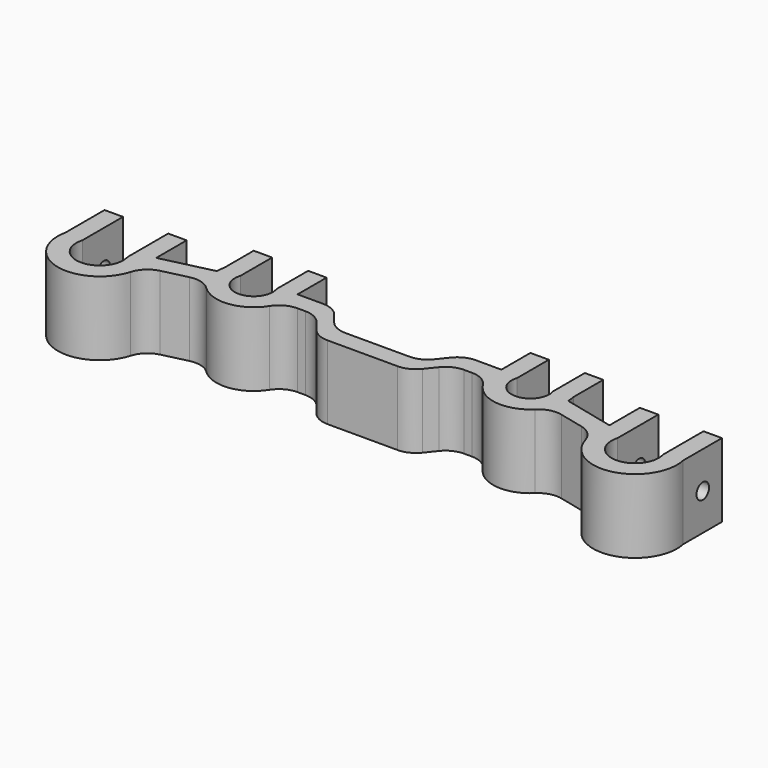
from build123d import *

# Parameters (mm, degrees)
F1_DEPTH = 16
F2_R     = 1.7
F3_DEPTH = 15.8
F4_DEPTH = 2
F5_R     = 1.7
F6_DEPTH = 17.8
F7_DEPTH = 2
F8_R     = 5


# Not quite as in the source:
# - a feature names something its author has since deleted; it is built from what else it names


with BuildPart() as f1:
    # F0 (on Top) → F1 (new body)
    with BuildSketch(Plane.XY):
        with BuildLine():
            ThreePointArc((-26.1, 1.2649110641), (-30, -4.1), (-33.9, 1.2649110641))
            Line((-33.9, 1.2649110641), (-33.9, 7.0992957397))
            ThreePointArc((-33.9, 7.0992957397), (-36.4699456608, 4.8733769756), (-37.9, 1.788854382))
            ThreePointArc((-37.9, 1.788854382), (-38.0425692419, 0.9628499311), (-38.0990116086, 0.1265344399))
            ThreePointArc((-38.0990116086, 0.1265344399), (-37.8794890645, -1.8771393349), (-37.1720292209, -3.7645712709))
            ThreePointArc((-37.1720292209, -3.7645712709), (-29.054976567, -8.0446833817), (-22.1507962187, -2))
            ThreePointArc((-22.1507962187, -2), (-21.9, 0), (-22.1507962187, 2))
            ThreePointArc((-22.1507962187, 2), (-23.5959659875, 4.9596722035), (-26.1, 7.0992957397))
            Line((-26.1, 7.0992957397), (-26.1, 1.2649110641))
        make_face()
        with BuildLine():
            ThreePointArc((-37.9, 1.788854382), (-36.4699456608, 4.8733769756), (-33.9, 7.0992957397))
            Line((-33.9, 7.0992957397), (-33.9, 9.8649110641))
            Line((-33.9, 9.8649110641), (-37.9, 9.8649110641))
            Line((-37.9, 9.8649110641), (-37.9, 1.788854382))
        make_face()
        with BuildLine():
            Line((-26.1, 9.8649110641), (-26.1, 7.0992957397))
            ThreePointArc((-26.1, 7.0992957397), (-23.5959659875, 4.9596722035), (-22.1507962187, 2))
            Line((-22.1507962187, 2), (-22.1, 2))
            Line((-22.1, 2), (-22.1, 9.8649110641))
            Line((-22.1, 9.8649110641), (-26.1, 9.8649110641))
        make_face()
        with BuildLine():
            Line((-22.1, 2), (-22.1507962187, 2))
            ThreePointArc((-22.1507962187, 2), (-21.9, 0), (-22.1507962187, -2))
            Line((-22.1507962187, -2), (-16.1507962187, -2))
            Line((-16.1507962187, -2), (-14.7945886775, -2))
            Line((-14.7945886775, -2), (-10, -8))
            Line((-10, -8), (0, -8))
            Line((0, -8), (0, -4))
            Line((0, -4), (-6, -4))
            Line((-6, -4), (-9.3562075412, -4))
            Line((-9.3562075412, -4), (-14.1507962187, 2))
            Line((-14.1507962187, 2), (-22.1, 2))
        make_face()
        with BuildLine():
            ThreePointArc((-37.1720292209, -3.7645712709), (-37.8794890645, -1.8771393349), (-38.0990116086, 0.1265344399))
            Line((-38.0990116086, 0.1265344399), (-49.14, -2.5037723523))
            Line((-49.14, -2.5037723523), (-49.14, -4.7826334039))
            ThreePointArc((-49.14, -4.7826334039), (-48.9961671585, -5.6705013446), (-48.9406864116, -6.5682314005))
            Line((-48.9406864116, -6.5682314005), (-37.1720292209, -3.7645712709))
        make_face()
        with BuildLine():
            Line((-49.14, -4.7826334039), (-49.14, -2.5037723523))
            Line((-49.14, -2.5037723523), (-49.8676687992, -2.6771256897))
            ThreePointArc((-49.8676687992, -2.6771256897), (-49.4391620268, -3.7075286109), (-49.14, -4.7826334039))
        make_face()
        with BuildLine():
            Line((-49.8676687992, -2.6771256897), (-49.14, -2.5037723523))
            Line((-49.14, -2.5037723523), (-49.14, 5.7342135624))
            Line((-49.14, 5.7342135624), (-53.14, 5.7342135624))
            Line((-53.14, 5.7342135624), (-53.14, 0.9881158051))
            ThreePointArc((-53.14, 0.9881158051), (-51.2517778793, -0.6194686338), (-49.8676687992, -2.6771256897))
        make_face()
        with BuildLine():
            ThreePointArc((-66.94, -4.7826334039), (-58.9383437694, -15.7355495952), (-48.9406864116, -6.5682314005))
            ThreePointArc((-48.9406864116, -6.5682314005), (-48.9961671585, -5.6705013446), (-49.14, -4.7826334039))
            ThreePointArc((-49.14, -4.7826334039), (-49.4391620268, -3.7075286109), (-49.8676687992, -2.6771256897))
            ThreePointArc((-49.8676687992, -2.6771256897), (-51.2517778793, -0.6194686338), (-53.14, 0.9881158051))
            Line((-53.14, 0.9881158051), (-53.14, -5.2657864376))
            ThreePointArc((-53.14, -5.2657864376), (-58.04, -11.78), (-62.94, -5.2657864376))
            Line((-62.94, -5.2657864376), (-62.94, 0.9881158051))
            ThreePointArc((-62.94, 0.9881158051), (-65.5189963637, -1.4959269496), (-66.94, -4.7826334039))
        make_face()
        with BuildLine():
            Line((-66.94, 5.7342135624), (-66.94, -4.7826334039))
            ThreePointArc((-66.94, -4.7826334039), (-65.5189963637, -1.4959269496), (-62.94, 0.9881158051))
            Line((-62.94, 0.9881158051), (-62.94, 5.7342135624))
            Line((-62.94, 5.7342135624), (-66.94, 5.7342135624))
        make_face()
    extrude(amount=F1_DEPTH)

    # F2 (on face) → F3 (cut, through all)
    with BuildSketch(Plane.YZ.offset(-22.1)):
        with Locations((5.2649110641, 8)):
            Circle(F2_R)
    extrude(amount=-F3_DEPTH, mode=Mode.SUBTRACT)

    # F2 (on face) → F4 (cut)
    with BuildSketch(Plane.YZ.offset(-22.1)):
        Polygon((8.1149110641, 6.3545517328), (8.1149110641, 9.6454482672), (5.2649110641, 11.2908965344), (2.4149110641, 9.6454482672), (2.4149110641, 6.3545517328), (5.2649110641, 4.7091034656), align=None)
        with Locations((5.2649110641, 8)):
            Circle(F2_R, mode=Mode.SUBTRACT)
    extrude(amount=-F4_DEPTH, mode=Mode.SUBTRACT)

    # F5 (on face) → F6 (cut, through all)
    with BuildSketch(Plane.YZ.offset(-49.14)):
        with Locations((0.5462276477, 8)):
            Circle(F5_R)
    extrude(amount=-F6_DEPTH, mode=Mode.SUBTRACT)

    # F5 (on face) → F7 (cut)
    with BuildSketch(Plane.YZ.offset(-49.14)):
        Polygon((3.3962276477, 6.3545517328), (3.3962276477, 9.6454482672), (0.5462276477, 11.2908965344), (-2.3037723523, 9.6454482672), (-2.3037723523, 6.3545517328), (0.5462276477, 4.7091034656), align=None)
        with Locations((0.5462276477, 8)):
            Circle(F5_R, mode=Mode.SUBTRACT)
    extrude(amount=-F7_DEPTH, mode=Mode.SUBTRACT)

    # F8
    f8_edges = [f1.edges().sort_by_distance(p)[0] for p in [
        (-48.940686, -6.568231, 8),
        (-37.172029, -3.764571, 8),
        (-22.150796, -2, 8),
        (-14.794589, -2, 8),
        (-10, -8, 8),
        (-9.356208, -4, 8),
        (-14.150796, 2, 8),
    ]]
    fillet(f8_edges, radius=F8_R)

    # F9: F1 across plane


with BuildPart() as f1_1:
    add(f1.part)
    add(f1.part.mirror(Plane.YZ))


solid = f1_1.part
